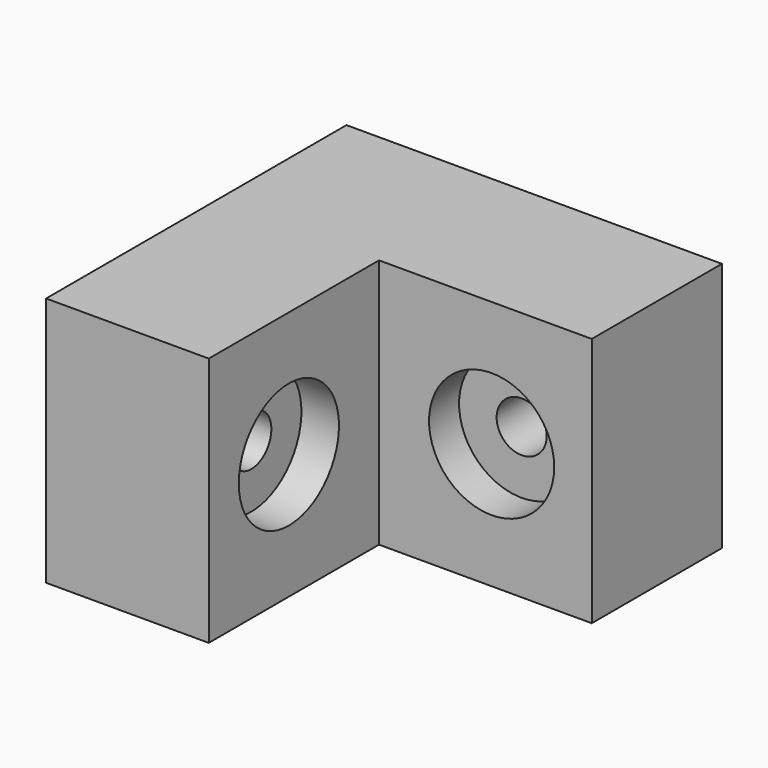
from build123d import *

# Parameters (mm, degrees)
F1_DEPTH = 20
F2_R     = 5
F3_DEPTH = 3
F4_R     = 2
F5_DEPTH = 10


# Not quite as in the source:
# - a pattern or mirror of a feature is missing from the dataset's text; its kind, count and spacing are read off the source's solid


with BuildPart() as f1:
    # F0 (on Top) → F1 (new body)
    with BuildSketch(Plane.XY):
        Polygon((30, 0), (0, 0), (0, -30), (13, -30), (13, -13), (30, -13), align=None)
    extrude(amount=F1_DEPTH)

    # F2 (on face) → F3 (cut)
    with BuildSketch(Plane.XZ.offset(13)):
        with Locations((22, 10)):
            Circle(F2_R)
    f3 = extrude(amount=-F3_DEPTH, mode=Mode.SUBTRACT)

    # F3_copies: F3 across plane
    add(f3.mirror(Plane(origin=(0, 0, 0), x_dir=(0.7071067812, -0.7071067812, 0), z_dir=(-0.7071067812, -0.7071067812, 0))), mode=Mode.SUBTRACT)

    # F4 (on face) → F5 (cut, through all)
    with BuildSketch(Plane.XZ.offset(10)):
        with Locations((22, 10)):
            Circle(F4_R)
    f5 = extrude(amount=-F5_DEPTH, mode=Mode.SUBTRACT)

    # F5_copies: F5 across plane
    add(f5.mirror(Plane(origin=(0, 0, 0), x_dir=(-0.7071067812, 0.7071067812, 0), z_dir=(-0.7071067812, -0.7071067812, 0))), mode=Mode.SUBTRACT)


solid = f1.part
